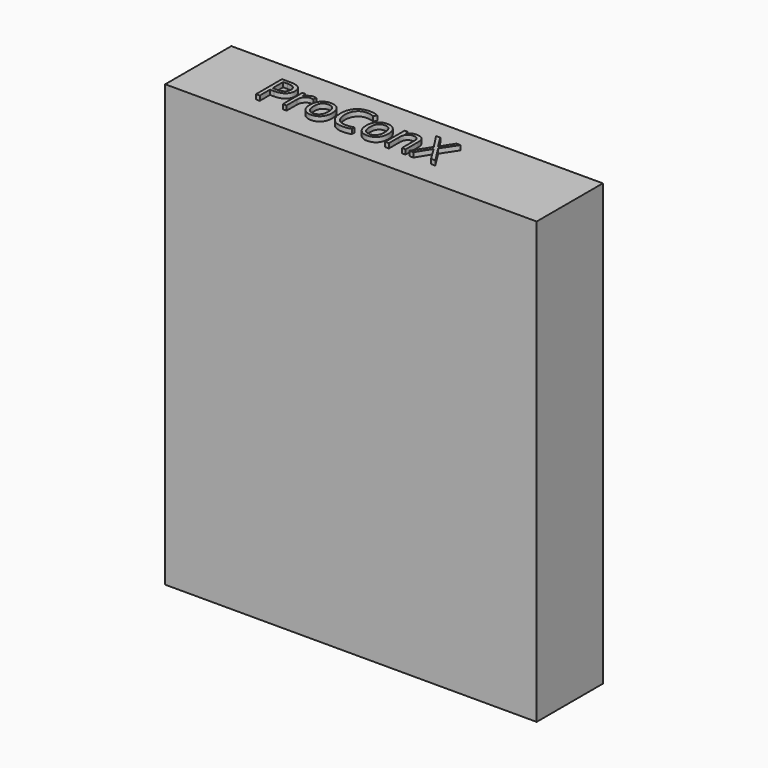
from build123d import *

# Parameters (mm, degrees)
F0_W         = 101.092
F0_H         = 22.5044
F1_DEPTH     = 119.888
F2_TEXT_SIZE = 12.3864675404
F3_DEPTH     = 1.27


# Not quite as in the source:
# - Text() gives the source's letters only with a copy of the font that has no kerning and outlines rounded to 1/6400 em; it was checked with that copy


with BuildPart() as f1:
    # F0 (on Top) → F1 (new body)
    with BuildSketch(Plane.XY):
        with Locations((8.2474797964, 0.5146493347)):
            Rectangle(F0_W, F0_H)
    extrude(amount=F1_DEPTH)

    # F2 (on face) → F3 (join)
    with BuildSketch(Plane.XY.offset(119.888)):
        with Locations((-24.0792920898, -4.1323275119)):
            Text('ProConX', F2_TEXT_SIZE, font='Open Sans', text_align=(TextAlign.LEFT, TextAlign.BOTTOM))
    extrude(amount=F3_DEPTH)


solid = f1.part
